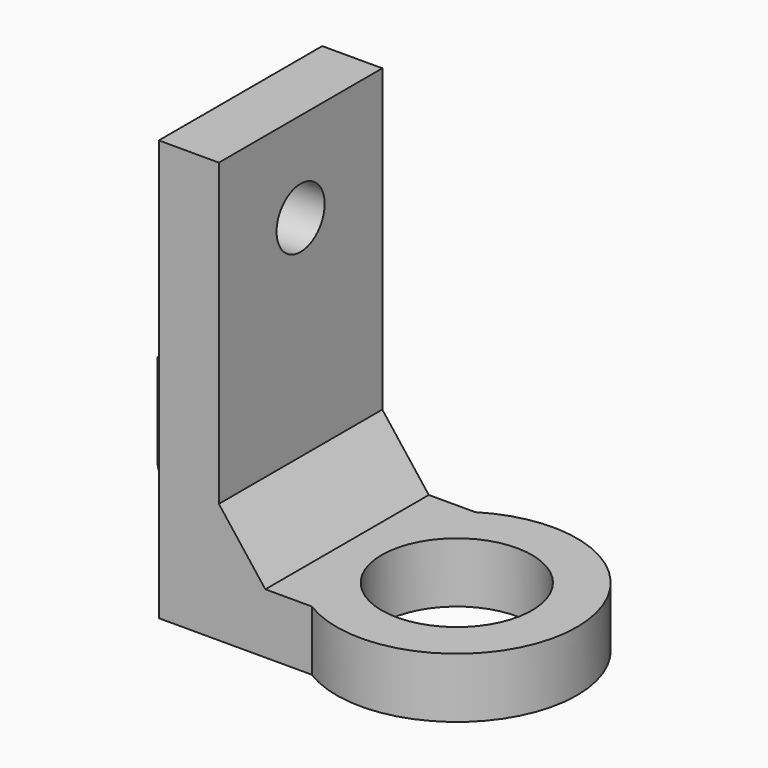
from build123d import *

# Parameters (mm, degrees)
F1_DEPTH    = 6.35
F0_W        = 3.175
F0_H        = 10.795
F2_DEPTH    = 44.45
F3_D        = 15.875
F5_D        = 6.35
F6_DEPTH    = 12.7
F7_T1_DEPTH = 14.2875
F9_DEPTH    = 21.59


# Not quite as in the source:
# - a fillet or chamfer that OpenCascade refuses, or shapes differently, is made with other operations: its cross-section is extruded or revolved along the edge and cut away or added


with BuildPart() as f1:
    # F0 (on Top) → F1 (new body)
    with BuildSketch(Plane.XY):
        with BuildLine():
            Line((22.86, 0), (16.1698598669, 0))
            ThreePointArc((16.1698598669, 0), (29.0375893482, -0.3012781979), (35.56, 10.795))
            ThreePointArc((35.56, 10.795), (29.0375893482, 21.8912781979), (16.1698598669, 21.59))
            Line((16.1698598669, 21.59), (22.86, 21.59))
            Line((22.86, 21.59), (22.86, 0))
        make_face()
        with BuildLine():
            ThreePointArc((16.1698598669, 21.59), (10.16, 10.795), (16.1698598669, 0))
            Line((16.1698598669, 0), (22.86, 0))
            Line((22.86, 0), (22.86, 21.59))
            Line((22.86, 21.59), (16.1698598669, 21.59))
        make_face()
        with BuildLine():
            Line((6.35, 10.795), (6.35, 0))
            Line((6.35, 0), (16.1698598669, 0))
            ThreePointArc((16.1698598669, 0), (10.16, 10.795), (16.1698598669, 21.59))
            Line((16.1698598669, 21.59), (6.35, 21.59))
            Line((6.35, 21.59), (6.35, 10.795))
        make_face()
    extrude(amount=F1_DEPTH)

    # F0 (on Top) → F2 (join)
    with BuildSketch(Plane.XY):
        with Locations((1.5875, 5.3975)):
            Rectangle(F0_W, F0_H)
        with Locations((4.7625, 5.3975)):
            Rectangle(F0_W, F0_H)
        with Locations((4.7625, 16.1925)):
            Rectangle(F0_W, F0_H)
        with Locations((1.5875, 16.1925)):
            Rectangle(F0_W, F0_H)
    extrude(amount=F2_DEPTH)

    # F3 (through all)
    with Locations(Plane(origin=(0, 0, 0), x_dir=(1, 0, 0), z_dir=(0, 0, -1))):
        with Locations((22.86, -10.795)):
            Hole(F3_D / 2)

    # F5 (through all)
    with Locations(Plane.YZ.offset(6.35)):
        with Locations((10.795, 34.925)):
            Hole(F5_D / 2)

    # F4 (on face) → F6 (join)
    with BuildSketch(Plane.YZ.offset(6.35)):
        Polygon((10.795, 12.7), (10.795, 19.05), (7.747, 19.05), (7.747, 6.35), (10.795, 6.35), align=None)
        Polygon((13.843, 19.05), (10.795, 19.05), (10.795, 12.7), (10.795, 6.35), (13.843, 6.35), align=None)
    extrude(amount=-F6_DEPTH)

    # F7: fillet of radius 3.175 on 2 edges, made by hand

    # F7_s2 → F7_t1 (cut)
    with BuildSketch(Plane.YZ.offset(-14.2875)):
        with BuildLine():
            ThreePointArc((10.922, 6.35), (8.6769359697, 7.2799359697), (7.747, 9.525))
            Line((7.747, 9.525), (7.747, 6.35))
            Line((7.747, 6.35), (10.922, 6.35))
        make_face()
        with BuildLine():
            ThreePointArc((13.843, 9.525), (12.9130640303, 7.2799359697), (10.668, 6.35))
            Line((10.668, 6.35), (13.843, 6.35))
            Line((13.843, 6.35), (13.843, 9.525))
        make_face()
    extrude(amount=F7_T1_DEPTH, mode=Mode.SUBTRACT)

    # F8 (on face) → F9 (join)
    with BuildSketch(Plane.XZ):
        Polygon((11.2599299335, 6.35), (6.35, 12.7), (6.35, 6.35), align=None)
    extrude(amount=-F9_DEPTH)


solid = f1.part
